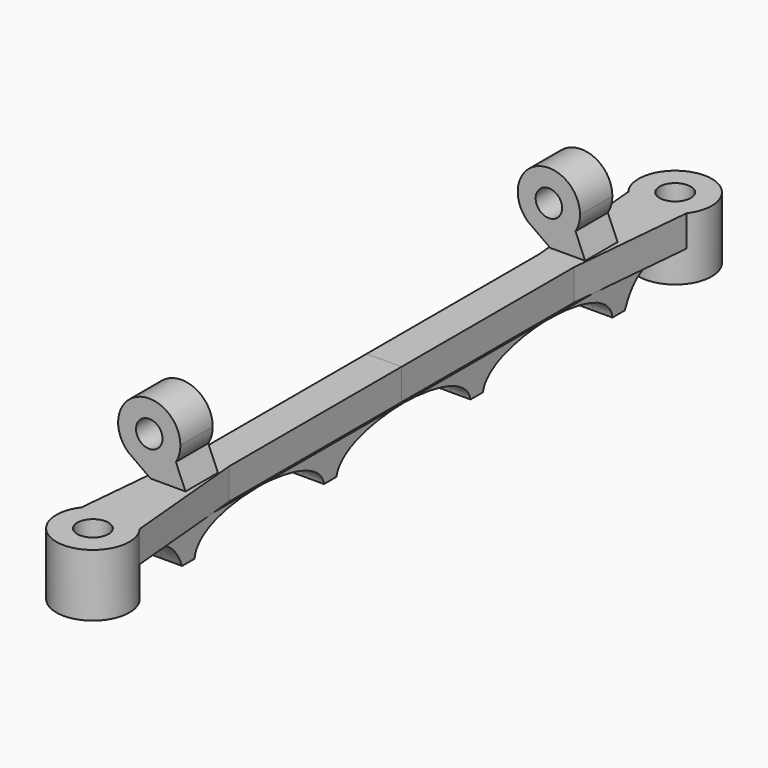
from build123d import *

# Parameters (mm, degrees)
F0_R     = 2
F1_DEPTH = 4
F3_START = -29.5
F2_R     = 1.7
F3_DEPTH = 5.2
F4_DEPTH = 4
F6_DEPTH = 2.5


# Not quite as in the source:
# - a feature names something its author has since deleted; it is built from what else it names


with BuildPart() as f1:
    # F0 (on Top) → F1 (new body)
    with BuildSketch(Plane.XY):
        with BuildLine():
            ThreePointArc((3.7401051407, 43.9236666505), (0, 42.07), (-3.7401051407, 43.9236666505))
            Line((-3.7401051407, 43.9236666505), (-2.25, 27.707760334))
            Line((-2.25, 27.707760334), (-2.25, 0))
            Line((-2.25, 0), (0, 0))
            Line((0, 0), (2.25, 0))
            Line((2.25, 0), (2.25, 27.707760334))
            Line((2.25, 27.707760334), (3.7401051407, 43.9236666505))
        make_face()
        with BuildLine():
            ThreePointArc((3.7401051407, 43.9236666505), (4.4535656592, 45.2680835845), (4.7, 46.77))
            ThreePointArc((4.7, 46.77), (-1.5019164155, 51.2235656592), (-3.7401051407, 43.9236666505))
            ThreePointArc((-3.7401051407, 43.9236666505), (0, 42.07), (3.7401051407, 43.9236666505))
        make_face()
        with Locations((0, 46.77)):
            Circle(F0_R, mode=Mode.SUBTRACT)
    extrude(amount=F1_DEPTH)

    # F2 (on Front) → F3 (join)
    with BuildSketch(Plane.XZ.offset(F3_START)):
        with BuildLine():
            Line((2.25, 4), (1.0056584573, 6.9262712577))
            ThreePointArc((1.0056584573, 6.9262712577), (-1.3823144995, 5.1355544295), (-4.3452027561, 5.4966289094))
            Line((-4.3452027561, 5.4966289094), (-2.25, 4))
            Line((-2.25, 4), (2.25, 4))
        make_face()
        with BuildLine():
            ThreePointArc((1.0056584573, 6.9262712577), (1.4375788293, 7.9234081388), (1.5851834752, 9))
            ThreePointArc((1.5851834752, 9), (-4.0346730574, 12.657330285), (-5.1028489317, 6.037824823))
            Line((-5.1028489317, 6.037824823), (-4.3452027561, 5.4966289094))
            ThreePointArc((-4.3452027561, 5.4966289094), (-1.3823144995, 5.1355544295), (1.0056584573, 6.9262712577))
        make_face()
        with Locations((-2.4148165248, 9)):
            Circle(F2_R, mode=Mode.SUBTRACT)
    extrude(amount=-F3_DEPTH)

    # F0 (on Top) → F4 (join)
    with BuildSketch(Plane.XY):
        with BuildLine():
            ThreePointArc((3.7401051407, 43.9236666505), (4.4535656592, 45.2680835845), (4.7, 46.77))
            ThreePointArc((4.7, 46.77), (-1.5019164155, 51.2235656592), (-3.7401051407, 43.9236666505))
            ThreePointArc((-3.7401051407, 43.9236666505), (0, 42.07), (3.7401051407, 43.9236666505))
        make_face()
        with Locations((0, 46.77)):
            Circle(F0_R, mode=Mode.SUBTRACT)
    extrude(amount=-F4_DEPTH)


with BuildPart() as f6:
    # F5 (on Right) → F6 (new body, symmetric)
    with BuildSketch(Plane.YZ):
        with BuildLine():
            Line((41.9037155807, 0), (35.57, 0))
            Line((35.57, 0), (35.57, -4))
            add(Edge.make_bspline(
                [(35.57, -4), (36.8272326887, -0.7868814864), (38.7368577904, 0), (41.9037155807, 0)],
                knots=[0, 0, 0, 0, 7.4910582068, 7.4910582068, 7.4910582068, 7.4910582068], degree=3))
        make_face()
        with BuildLine():
            Line((35.57, -4), (35.57, 0))
            Line((35.57, 0), (23.2577491552, 0))
            add(Edge.make_bspline(
                [(23.2577491552, 0), (27.2780284286, 0), (33.1432744861, -0.8353546145), (33.57, -4)],
                knots=[0, 0, 0, 0, 11.0608551879, 11.0608551879, 11.0608551879, 11.0608551879], degree=3))
            Line((33.57, -4), (35.57, -4))
        make_face()
    extrude(amount=F6_DEPTH, both=True)


with BuildPart() as f6b:
    # F5 (on Right) → F6, piece 2 (new body, symmetric)
    with BuildSketch(Plane.YZ):
        with BuildLine():
            add(Edge.make_bspline(
                [(12.77, -4), (13.317771256, -0.9807739407), (19.7162237018, 0), (23.2577491552, 0)],
                knots=[0, 0, 0, 0, 11.2246551101, 11.2246551101, 11.2246551101, 11.2246551101], degree=3))
            Line((23.2577491552, 0), (0, 0))
            add(Edge.make_bspline(
                [(10.77, -4), (10.1670185104, -0.9323008708), (3.7685674615, 0), (0, 0)],
                knots=[0, 0, 0, 0, 11.4888163011, 11.4888163011, 11.4888163011, 11.4888163011], degree=3))
            Line((10.77, -4), (12.77, -4))
        make_face()
    extrude(amount=F6_DEPTH, both=True)


with BuildPart() as f7_1:
    # F7: instance of F1
    add(f1.part.mirror(Plane(origin=(0, 0, 2), x_dir=(1, 0, 0), z_dir=(0, -1, 0))))


with BuildPart() as f7_2:
    # F7: instance of F6
    add(f6.part.mirror(Plane(origin=(0, 0, 2), x_dir=(1, 0, 0), z_dir=(0, -1, 0))))


with BuildPart() as f7_3:
    # F7: instance of F6b
    add(f6b.part.mirror(Plane(origin=(0, 0, 2), x_dir=(1, 0, 0), z_dir=(0, -1, 0))))


solid = Compound([f1.part, f6.part, f6b.part, f7_1.part, f7_2.part, f7_3.part])
